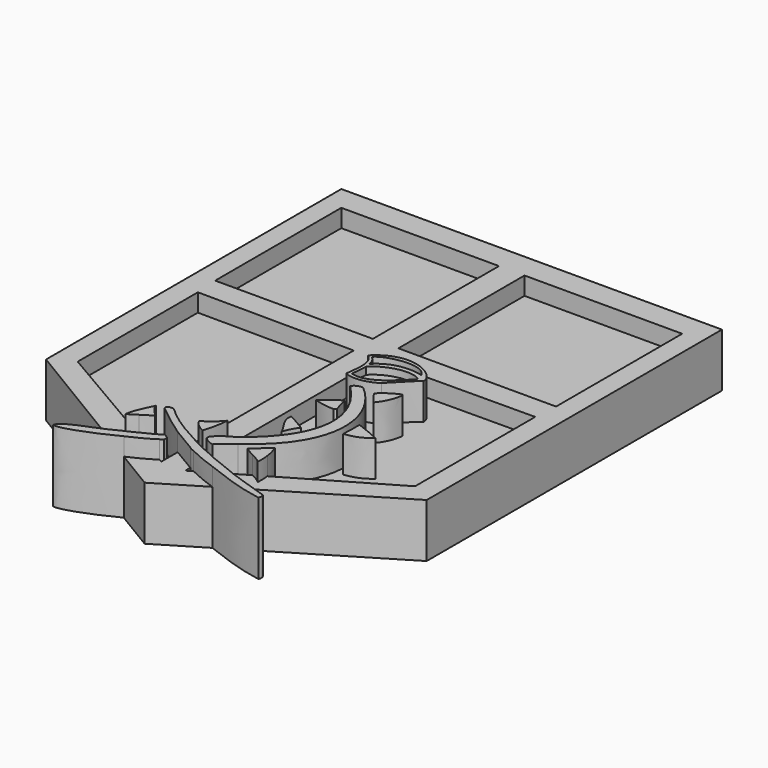
from build123d import *

# Parameters (mm, degrees)
F1_DEPTH = 3.81
F0_W     = 11.176
F0_H     = 11.176
F2_DEPTH = 2.54
F3_DEPTH = 5.08
F4_DEPTH = 4.572


with BuildPart() as f1:
    # F0 (on Top) → F1 (new body)
    with BuildSketch(Plane.XY):
        with BuildLine():
            add(Edge.make_bspline(
                [(1.7478264633, -8.0203386829), (2.3949102033, -7.7400864102), (3.0131435487, -7.4116708711), (3.5160593419, -7.0720952225)],
                knots=[0, 0, 0, 0, 2.0064429155, 2.0064429155, 2.0064429155, 2.0064429155], degree=3))
            Line((1.7478264633, -8.0203386829), (4.6047386499, -9.7420183434))
            Line((4.6047386499, -9.7420183434), (7.8442137424, -7.789792299))
            add(Edge.make_bspline(
                [(5.8583344234, -6.9758380503), (6.5180123784, -7.3072281666), (7.161768619, -7.5551345944), (7.8442137424, -7.789792299)],
                knots=[0, 0, 0, 0, 2.1462148514, 2.1462148514, 2.1462148514, 2.1462148514], degree=3))
            Line((5.8583344234, -6.9758380503), (5.4626313076, -7.2067989968))
            Line((5.4626313076, -7.2067989968), (5.4626313076, -6.7658983171))
            Line((5.4626313076, -6.7658983171), (3.7468459923, -5.7425037958))
            Line((3.7468459923, -5.7425037958), (3.7468459923, -6.668202544))
            Line((3.7468459923, -6.668202544), (3.9543234743, -6.8065118976))
            Line((3.9543234743, -6.8065118976), (3.7468459923, -6.932241008))
            Line((3.7468459923, -6.932241008), (3.7468459923, -7.2067989968))
            Line((3.7468459923, -7.2067989968), (3.5160593419, -7.0720952225))
        make_face()
        Polygon((3.7468459923, -6.668202544), (3.7468459923, -6.932241008), (3.9543234743, -6.8065118976), align=None)
    extrude(amount=F1_DEPTH)



with BuildPart() as f1b:
    # F0 (on Top) → F1, piece 2 (new body)
    with BuildSketch(Plane.XY):
        with BuildLine():
            Line((18.0921386499, 24.5479816566), (-8.8826613501, 24.5479816566))
            Line((-8.8826613501, 24.5479816566), (-8.8826613501, -1.6140183434))
            Line((-8.8826613501, -1.6140183434), (1.1086808245, -7.6351661699))
            add(Edge.make_bspline(
                [(2.9416688976, -6.7368394326), (2.373174997, -7.0127416402), (1.7493715277, -7.3646083474), (1.1086808245, -7.6351661699)],
                knots=[0, 0, 0, 0, 2.0412829797, 2.0412829797, 2.0412829797, 2.0412829797], degree=3))
            Line((2.9416688976, -6.7368394326), (0.7978946411, -5.4855777885))
            add(Edge.make_bspline(
                [(0.7978946411, -5.4855777885), (0.5607364427, -5.6443807503), (0.3392614036, -5.7966192163), (0.1594885398, -5.8946078643)],
                knots=[0.8541472288, 0.8541472288, 0.8541472288, 0.8541472288, 1.6626558138, 1.6626558138, 1.6626558138, 1.6626558138], degree=3))
            add(Edge.make_bspline(
                [(0.1594885398, -5.8946078643), (0.1844977105, -5.6643810778), (0.2451815779, -5.4372146163), (0.3267234324, -5.210568207)],
                knots=[0, 0, 0, 0, 0.730730804, 0.730730804, 0.730730804, 0.730730804], degree=3))
            Line((0.3267234324, -5.210568207), (-7.3511232622, -0.7292217924))
            Line((-7.3511232622, -0.7292217924), (-7.3511232622, 9.9187362939))
            Line((-7.3511232622, 9.9187362939), (3.7468459923, 9.8566794768))
            Line((3.7468459923, 9.8566794768), (3.7468459923, -5.1428475417))
            Line((3.7468459923, -5.1428475417), (5.4626313076, -6.1111301184))
            Line((5.4626313076, -6.1111301184), (5.4626313076, -5.3286819914))
            add(Edge.make_bspline(
                [(5.4626313076, -5.3286819914), (5.4171880556, -5.2900749749), (5.3747972554, -5.2519792783), (5.3360559978, -5.2162380889)],
                knots=[0.7997569786, 0.7997569786, 0.7997569786, 0.7997569786, 0.9823963323, 0.9823963323, 0.9823963323, 0.9823963323], degree=3))
            add(Edge.make_bspline(
                [(5.4626313076, -5.0888806677), (5.4209392766, -5.1307410959), (5.3789487872, -5.173187785), (5.3360559978, -5.2162380889)],
                knots=[1.4886530847, 1.4886530847, 1.4886530847, 1.4886530847, 1.6788346934, 1.6788346934, 1.6788346934, 1.6788346934], degree=3))
            Line((5.4626313076, -5.0888806677), (5.4626313076, 9.8566794768))
            Line((5.4626313076, 9.8566794768), (16.5606005621, 9.9187362939))
            Line((16.5606005621, 9.9187362939), (16.5606005621, -0.7292217924))
            Line((16.5606005621, -0.7292217924), (9.4219063748, -4.8958798247))
            add(Edge.make_bspline(
                [(9.4498144463, -5.7773548178), (9.4676312637, -5.4715193492), (9.4601174375, -5.1821135329), (9.4219063748, -4.8958798247)],
                knots=[0, 0, 0, 0, 0.8835893602, 0.8835893602, 0.8835893602, 0.8835893602], degree=3))
            add(Edge.make_bspline(
                [(8.7163211778, -5.3077103572), (8.9863336594, -5.4468521573), (9.2526252745, -5.5869770135), (9.4498144463, -5.7773548178)],
                knots=[0.7875820287, 0.7875820287, 0.7875820287, 0.7875820287, 1.6683513681, 1.6683513681, 1.6683513681, 1.6683513681], degree=3))
            Line((8.7163211778, -5.3077103572), (6.5198496095, -6.5897299623))
            add(Edge.make_bspline(
                [(8.467863043, -7.4139584455), (7.7391685918, -7.1327229962), (7.1244202554, -6.8972771987), (6.5198496095, -6.5897299623)],
                knots=[0, 0, 0, 0, 2.1152089565, 2.1152089565, 2.1152089565, 2.1152089565], degree=3))
            Line((8.467863043, -7.4139584455), (18.0921386499, -1.6140183434))
            Line((18.0921386499, -1.6140183434), (18.0921386499, 24.5479816566))
        make_face()
        with BuildLine():
            add(Edge.make_bspline(
                [(4.7253458761, -4.7482554801), (4.3430225924, -4.5879259706), (3.9915316738, -4.3042670004), (3.8743680343, -3.9959414862)],
                knots=[0, 0, 0, 0, 1.1358431373, 1.1358431373, 1.1358431373, 1.1358431373], degree=3))
            add(Edge.make_bspline(
                [(3.8743680343, -3.9959414862), (4.3306895532, -3.7122820504), (4.7253458761, -3.403956769), (5.0706705078, -2.9723013286)],
                knots=[0, 0, 0, 0, 1.5744773039, 1.5744773039, 1.5744773039, 1.5744773039], degree=3))
            add(Edge.make_bspline(
                [(5.0706705078, -2.9723013286), (5.0213383511, -3.5827853717), (4.9041747116, -4.1809366085), (4.7253458761, -4.7482554801)],
                knots=[0, 0, 0, 0, 1.8092159212, 1.8092159212, 1.8092159212, 1.8092159212], degree=3))
        make_face(mode=Mode.SUBTRACT)
        with Locations((-1.888773113, 17.1971733798)):
            Rectangle(F0_W, F0_H, mode=Mode.SUBTRACT)
        with Locations((11.0982504129, 17.1971733798)):
            Rectangle(F0_W, F0_H, mode=Mode.SUBTRACT)
        with BuildLine():
            add(Edge.make_bspline(
                [(5.4626313076, -5.3286819914), (5.4171880556, -5.2900749749), (5.3747972554, -5.2519792783), (5.3360559978, -5.2162380889)],
                knots=[0.7997569786, 0.7997569786, 0.7997569786, 0.7997569786, 0.9823963323, 0.9823963323, 0.9823963323, 0.9823963323], degree=3))
            Line((5.4626313076, -5.3286819914), (5.4626313076, -5.0888806677))
            add(Edge.make_bspline(
                [(5.4626313076, -5.0888806677), (5.4209392766, -5.1307410959), (5.3789487872, -5.173187785), (5.3360559978, -5.2162380889)],
                knots=[1.4886530847, 1.4886530847, 1.4886530847, 1.4886530847, 1.6788346934, 1.6788346934, 1.6788346934, 1.6788346934], degree=3))
        make_face()
    extrude(amount=F1_DEPTH)


with BuildPart() as f1_1:
    add(f1.part)

    add(f1b.part)  # F2 merges F1b
    # F0 (on Top) → F2 (join)
    with BuildSketch(Plane.XY):
        with BuildLine():
            Line((0.7978946411, -5.4855777885), (2.9416688976, -6.7368394326))
            Line((2.9416688976, -6.7368394326), (3.4156478941, -6.4474181272))
            Line((3.4156478941, -6.4474181272), (3.7468459923, -6.668202544))
            Line((3.7468459923, -6.668202544), (3.7468459923, -5.7425037958))
            add(Edge.make_bspline(
                [(3.7468459923, -5.7425037958), (2.9118994717, -5.1698186435), (2.13727355, -4.5987805352), (1.3940667268, -3.9734384045)],
                knots=[0, 0, 0, 0, 2.9436648299, 2.9436648299, 2.9436648299, 2.9436648299], degree=3))
            add(Edge.make_bspline(
                [(1.3940667268, -3.9734384045), (1.3278889237, -3.6056702957), (1.8194783479, -3.6950502545), (1.8866790924, -3.7452809047)],
                knots=[0, 0, 0, 0, 0.5428837698, 0.5428837698, 0.5428837698, 0.5428837698], degree=3))
            add(Edge.make_bspline(
                [(1.8866790924, -3.7452809047), (2.3712625261, -4.2291865684), (3.0714494642, -4.7257412225), (3.7468459923, -5.1428475417)],
                knots=[0, 0, 0, 0, 2.3266743219, 2.3266743219, 2.3266743219, 2.3266743219], degree=3))
            Line((3.7468459923, -5.1428475417), (3.7468459923, 9.8566794768))
            Line((3.7468459923, 9.8566794768), (-7.3511232622, 9.9187362939))
            Line((-7.3511232622, 9.9187362939), (-7.3511232622, -0.7292217924))
            Line((-7.3511232622, -0.7292217924), (0.3267234324, -5.210568207))
            add(Edge.make_bspline(
                [(0.3267234324, -5.210568207), (0.4654459663, -4.8249875208), (0.6645362865, -4.4409119844), (0.8510400658, -4.0458338335)],
                knots=[0.730730804, 0.730730804, 0.730730804, 0.730730804, 1.973881691, 1.973881691, 1.973881691, 1.973881691], degree=3))
            add(Edge.make_bspline(
                [(1.5713630245, -5.0165219947), (1.2786596781, -4.7041471116), (0.9113978012, -4.3504554778), (0.8510400658, -4.0458338335)],
                knots=[0, 0, 0, 0, 1.2087599726, 1.2087599726, 1.2087599726, 1.2087599726], degree=3))
            add(Edge.make_bspline(
                [(1.5713630245, -5.0165219947), (1.316488917, -5.1427171478), (1.0484399312, -5.3178107267), (0.7978946411, -5.4855777885)],
                knots=[0, 0, 0, 0, 0.8541472288, 0.8541472288, 0.8541472288, 0.8541472288], degree=3))
        make_face()
        with BuildLine():
            add(Edge.make_bspline(
                [(5.4626313076, -6.1111301184), (5.7463049889, -6.248251535), (6.1555313878, -6.4591150731), (6.5198496095, -6.5897299623)],
                knots=[0, 0, 0, 0, 1.1605034892, 1.1605034892, 1.1605034892, 1.1605034892], degree=3))
            Line((6.5198496095, -6.5897299623), (8.7163211778, -5.3077103572))
            add(Edge.make_bspline(
                [(8.0298092216, -4.9015800469), (8.2304568628, -5.0596558086), (8.4748766036, -5.1832900621), (8.7163211778, -5.3077103572)],
                knots=[0, 0, 0, 0, 0.7875820287, 0.7875820287, 0.7875820287, 0.7875820287], degree=3))
            add(Edge.make_bspline(
                [(9.1535774991, -3.8841355126), (8.725322783, -4.1867932305), (8.3324862644, -4.7373720445), (8.0298092216, -4.9015800469)],
                knots=[0, 0, 0, 0, 1.5159315689, 1.5159315689, 1.5159315689, 1.5159315689], degree=3))
            add(Edge.make_bspline(
                [(9.4219063748, -4.8958798247), (9.3772484403, -4.561353504), (9.290661138, -4.2311599671), (9.1535774991, -3.8841355126)],
                knots=[0.8835893602, 0.8835893602, 0.8835893602, 0.8835893602, 1.916255637, 1.916255637, 1.916255637, 1.916255637], degree=3))
            Line((9.4219063748, -4.8958798247), (16.5606005621, -0.7292217924))
            Line((16.5606005621, -0.7292217924), (16.5606005621, 9.9187362939))
            Line((16.5606005621, 9.9187362939), (5.4626313076, 9.8566794768))
            Line((5.4626313076, 9.8566794768), (5.4626313076, -5.0888806677))
            add(Edge.make_bspline(
                [(6.6764084622, -4.2053270154), (6.0970362861, -4.4694731571), (5.7889771144, -4.7612167258), (5.4626313076, -5.0888806677)],
                knots=[0, 0, 0, 0, 1.4886530847, 1.4886530847, 1.4886530847, 1.4886530847], degree=3))
            add(Edge.make_bspline(
                [(7.7819717117, 4.5010265894), (11.7669496685, 0.5076405359), (8.4563568234, -2.8782894369), (6.6764084622, -4.2053270154)],
                knots=[0, 0, 0, 0, 8.7762670419, 8.7762670419, 8.7762670419, 8.7762670419], degree=3))
            add(Edge.make_bspline(
                [(8.4548452869, 4.8108319752), (8.1331767142, 4.8204651102), (7.9173492268, 4.7341338359), (7.7819717117, 4.5010265894)],
                knots=[0, 0, 0, 0, 0.7407686719, 0.7407686719, 0.7407686719, 0.7407686719], degree=3))
            add(Edge.make_bspline(
                [(7.2531360202, -4.7906204127), (11.5543589927, -1.8333768239), (11.3695440814, 2.3211010266), (8.4548452869, 4.8108319752)],
                knots=[0, 0, 0, 0, 9.6763625975, 9.6763625975, 9.6763625975, 9.6763625975], degree=3))
            add(Edge.make_bspline(
                [(7.2531360202, -4.7906204127), (6.8616638891, -5.0828703679), (6.516339723, -5.3418637253), (6.18505897, -5.7105016895)],
                knots=[0, 0, 0, 0, 1.4095992865, 1.4095992865, 1.4095992865, 1.4095992865], degree=3))
            add(Edge.make_bspline(
                [(6.18505897, -5.7105016895), (5.9191426632, -5.6765978446), (5.6616221447, -5.4977377299), (5.4626313076, -5.3286819914)],
                knots=[0, 0, 0, 0, 0.7997569786, 0.7997569786, 0.7997569786, 0.7997569786], degree=3))
            Line((5.4626313076, -5.3286819914), (5.4626313076, -6.1111301184))
        make_face()
        with BuildLine():
            add(Edge.make_bspline(
                [(8.2225874066, -2.1199558396), (7.980666589, -1.5371904301), (7.3776016943, -1.06202811), (7.4968249537, -0.3716596111)],
                knots=[0, 0, 0, 0, 1.892952942, 1.892952942, 1.892952942, 1.892952942], degree=3))
            add(Edge.make_bspline(
                [(7.4968249537, -0.3716596111), (7.9144071788, -0.5795955658), (8.3382222801, -0.8238631417), (8.7610548362, -1.0945518734)],
                knots=[0, 0, 0, 0, 1.4563139836, 1.4563139836, 1.4563139836, 1.4563139836], degree=3))
            add(Edge.make_bspline(
                [(8.7610548362, -1.0945518734), (8.5307387635, -1.3888530666), (8.3580762148, -1.7526769079), (8.2225874066, -2.1199558396)],
                knots=[0, 0, 0, 0, 1.1581884418, 1.1581884418, 1.1581884418, 1.1581884418], degree=3))
        make_face(mode=Mode.SUBTRACT)
        with BuildLine():
            add(Edge.make_bspline(
                [(7.3553556576, 2.0199252758), (7.7547212131, 2.3667903151), (8.1656808034, 2.7087128256), (8.6129242554, 2.9652146623)],
                knots=[0, 0, 0, 0, 1.5732294182, 1.5732294182, 1.5732294182, 1.5732294182], degree=3))
            add(Edge.make_bspline(
                [(8.6129242554, 2.9652146623), (8.7030185387, 2.6003564708), (8.7855923921, 2.2661380935), (8.924013935, 1.8957672874)],
                knots=[0, 0, 0, 0, 1.1137748769, 1.1137748769, 1.1137748769, 1.1137748769], degree=3))
            add(Edge.make_bspline(
                [(8.924013935, 1.8957672874), (8.8682854548, 1.8838609103), (8.8227195665, 1.8443046138), (8.7929395959, 1.7774439184)],
                knots=[0, 0, 0, 0, 0.1765811486, 0.1765811486, 0.1765811486, 0.1765811486], degree=3))
            add(Edge.make_bspline(
                [(8.7929395959, 1.7774439184), (8.2995798439, 1.7669230001), (7.7650537714, 1.8754522316), (7.3553556576, 2.0199252758)],
                knots=[0, 0, 0, 0, 1.4578905268, 1.4578905268, 1.4578905268, 1.4578905268], degree=3))
        make_face(mode=Mode.SUBTRACT)
        with BuildLine():
            add(Edge.make_bspline(
                [(9.3703940511, 4.657026846), (9.526329115, 4.3411930092), (9.7634745762, 4.0558967739), (10.0183784962, 3.7871007808)],
                knots=[0, 0, 0, 0, 1.0847373876, 1.0847373876, 1.0847373876, 1.0847373876], degree=3))
            add(Edge.make_bspline(
                [(10.647803545, 5.5152899586), (10.1649090648, 5.3156521171), (9.7082797438, 5.0143827684), (9.3703940511, 4.657026846)],
                knots=[0, 0, 0, 0, 1.5389576296, 1.5389576296, 1.5389576296, 1.5389576296], degree=3))
            add(Edge.make_bspline(
                [(10.7278358191, 5.4443958215), (10.7111549005, 5.483365152), (10.6785837561, 5.5158259347), (10.647803545, 5.5152899586)],
                knots=[0, 0, 0, 0, 0.1069165262, 0.1069165262, 0.1069165262, 0.1069165262], degree=3))
            add(Edge.make_bspline(
                [(10.0183784962, 3.7871007808), (10.3937508538, 4.238513764), (10.6756044552, 4.798698239), (10.7278358191, 5.4443958215)],
                knots=[0, 0, 0, 0, 1.8027635855, 1.8027635855, 1.8027635855, 1.8027635855], degree=3))
        make_face(mode=Mode.SUBTRACT)
        with BuildLine():
            add(Edge.make_bspline(
                [(11.0556203872, -0.2232317202), (11.1070927233, 0.2977081749), (11.0771935433, 0.7693253574), (11.0852858052, 1.1983034201)],
                knots=[0, 0, 0, 0, 1.4218446441, 1.4218446441, 1.4218446441, 1.4218446441], degree=3))
            add(Edge.make_bspline(
                [(11.0852858052, 1.1983034201), (11.5990201011, 0.9836831596), (12.2310789302, 0.7833028212), (12.762288563, 0.5076405359)],
                knots=[0, 0, 0, 0, 1.813657484, 1.813657484, 1.813657484, 1.813657484], degree=3))
            add(Edge.make_bspline(
                [(12.762288563, 0.5076405359), (12.3673435301, 0.1413055725), (11.8517661467, -0.1177676531), (11.0556203872, -0.2232317202)],
                knots=[0, 0, 0, 0, 1.8565803287, 1.8565803287, 1.8565803287, 1.8565803287], degree=3))
        make_face(mode=Mode.SUBTRACT)
        with BuildLine():
            add(Edge.make_bspline(
                [(6.2449835241, 7.9964315519), (7.0174927823, 7.4354913086), (6.7296018824, 6.3399062492), (6.6649555229, 5.5675776675)],
                knots=[0, 0, 0, 0, 2.4648950629, 2.4648950629, 2.4648950629, 2.4648950629], degree=3))
            add(Edge.make_bspline(
                [(10.5703761801, 7.6710619032), (10.2531649172, 8.6557241157), (8.0357557163, 9.7695672885), (6.2449835241, 7.9964315519)],
                knots=[0, 0, 0, 0, 4.3376130576, 4.3376130576, 4.3376130576, 4.3376130576], degree=3))
            add(Edge.make_bspline(
                [(10.5871027336, 7.5067980215), (10.5815272157, 7.5615526487), (10.5759516979, 7.616307276), (10.5703761801, 7.6710619032)],
                knots=[0, 0, 0, 0, 0.1651132958, 0.1651132958, 0.1651132958, 0.1651132958], degree=3))
            add(Edge.make_bspline(
                [(8.9133325964, 5.8710686862), (9.5503591001, 6.4451182261), (10.0034726784, 7.0829736069), (10.5871027336, 7.5067980215)],
                knots=[0, 0, 0, 0, 2.3403241079, 2.3403241079, 2.3403241079, 2.3403241079], degree=3))
            add(Edge.make_bspline(
                [(6.6649555229, 5.5675776675), (6.9833141752, 5.3194463253), (8.069335483, 5.2957138978), (8.9133325964, 5.8710686862)],
                knots=[0, 0, 0, 0, 2.2687675649, 2.2687675649, 2.2687675649, 2.2687675649], degree=3))
        make_face(mode=Mode.SUBTRACT)
        with BuildLine():
            Line((5.4626313076, -7.2067989968), (5.8583344234, -6.9758380503))
            add(Edge.make_bspline(
                [(5.8583344234, -6.9758380503), (5.6914929301, -6.9214603864), (5.567043554, -6.8462723866), (5.4626313076, -6.7658983171)],
                knots=[0, 0, 0, 0, 0.4479460319, 0.4479460319, 0.4479460319, 0.4479460319], degree=3))
            Line((5.4626313076, -6.7658983171), (5.4626313076, -7.2067989968))
        make_face()
        with Locations((-1.888773113, 17.1971733798)):
            Rectangle(F0_W, F0_H)
        with Locations((11.0982504129, 17.1971733798)):
            Rectangle(F0_W, F0_H)
    extrude(amount=F2_DEPTH)

    # F0 (on Top) → F3 (join)
    with BuildSketch(Plane.XY):
        with BuildLine():
            Line((0.3267234324, -5.210568207), (0.7978946411, -5.4855777885))
            add(Edge.make_bspline(
                [(1.5713630245, -5.0165219947), (1.316488917, -5.1427171478), (1.0484399312, -5.3178107267), (0.7978946411, -5.4855777885)],
                knots=[0, 0, 0, 0, 0.8541472288, 0.8541472288, 0.8541472288, 0.8541472288], degree=3))
            add(Edge.make_bspline(
                [(1.5713630245, -5.0165219947), (1.2786596781, -4.7041471116), (0.9113978012, -4.3504554778), (0.8510400658, -4.0458338335)],
                knots=[0, 0, 0, 0, 1.2087599726, 1.2087599726, 1.2087599726, 1.2087599726], degree=3))
            add(Edge.make_bspline(
                [(0.3267234324, -5.210568207), (0.4654459663, -4.8249875208), (0.6645362865, -4.4409119844), (0.8510400658, -4.0458338335)],
                knots=[0.730730804, 0.730730804, 0.730730804, 0.730730804, 1.973881691, 1.973881691, 1.973881691, 1.973881691], degree=3))
        make_face()
        with BuildLine():
            add(Edge.make_bspline(
                [(0.7978946411, -5.4855777885), (0.5607364427, -5.6443807503), (0.3392614036, -5.7966192163), (0.1594885398, -5.8946078643)],
                knots=[0.8541472288, 0.8541472288, 0.8541472288, 0.8541472288, 1.6626558138, 1.6626558138, 1.6626558138, 1.6626558138], degree=3))
            Line((0.7978946411, -5.4855777885), (0.3267234324, -5.210568207))
            add(Edge.make_bspline(
                [(0.1594885398, -5.8946078643), (0.1844977105, -5.6643810778), (0.2451815779, -5.4372146163), (0.3267234324, -5.210568207)],
                knots=[0, 0, 0, 0, 0.730730804, 0.730730804, 0.730730804, 0.730730804], degree=3))
        make_face()
        with BuildLine():
            Line((1.7478264633, -8.0203386829), (1.1086808245, -7.6351661699))
            add(Edge.make_bspline(
                [(-2.1559654269, -9.3924161047), (-1.9764574245, -8.7245535105), (0.0426645383, -8.2730045542), (1.1086808245, -7.6351661699)],
                knots=[0, 0, 0, 0, 3.7075386013, 3.7075386013, 3.7075386013, 3.7075386013], degree=3))
            add(Edge.make_bspline(
                [(1.7478264633, -8.0203386829), (0.5305836094, -8.6686918512), (-1.6694880323, -9.5958048478), (-2.1559654269, -9.3924161047)],
                knots=[0, 0, 0, 0, 4.1378965155, 4.1378965155, 4.1378965155, 4.1378965155], degree=3))
        make_face()
        with BuildLine():
            add(Edge.make_bspline(
                [(2.9416688976, -6.7368394326), (2.373174997, -7.0127416402), (1.7493715277, -7.3646083474), (1.1086808245, -7.6351661699)],
                knots=[0, 0, 0, 0, 2.0412829797, 2.0412829797, 2.0412829797, 2.0412829797], degree=3))
            Line((1.1086808245, -7.6351661699), (1.7478264633, -8.0203386829))
            add(Edge.make_bspline(
                [(1.7478264633, -8.0203386829), (2.3949102033, -7.7400864102), (3.0131435487, -7.4116708711), (3.5160593419, -7.0720952225)],
                knots=[0, 0, 0, 0, 2.0064429155, 2.0064429155, 2.0064429155, 2.0064429155], degree=3))
            Line((3.5160593419, -7.0720952225), (2.9416688976, -6.7368394326))
        make_face()
        Polygon((3.4156478941, -6.4474181272), (2.9416688976, -6.7368394326), (3.5160593419, -7.0720952225), (3.7468459923, -6.932241008), (3.7468459923, -6.668202544), align=None)
        Polygon((5.4626313076, -6.7658983171), (5.4626313076, -6.1111301184), (3.7468459923, -5.1428475417), (3.7468459923, -5.7425037958), align=None)
        with BuildLine():
            Line((3.7468459923, -5.7425037958), (3.7468459923, -5.1428475417))
            add(Edge.make_bspline(
                [(1.8866790924, -3.7452809047), (2.3712625261, -4.2291865684), (3.0714494642, -4.7257412225), (3.7468459923, -5.1428475417)],
                knots=[0, 0, 0, 0, 2.3266743219, 2.3266743219, 2.3266743219, 2.3266743219], degree=3))
            add(Edge.make_bspline(
                [(1.3940667268, -3.9734384045), (1.3278889237, -3.6056702957), (1.8194783479, -3.6950502545), (1.8866790924, -3.7452809047)],
                knots=[0, 0, 0, 0, 0.5428837698, 0.5428837698, 0.5428837698, 0.5428837698], degree=3))
            add(Edge.make_bspline(
                [(3.7468459923, -5.7425037958), (2.9118994717, -5.1698186435), (2.13727355, -4.5987805352), (1.3940667268, -3.9734384045)],
                knots=[0, 0, 0, 0, 2.9436648299, 2.9436648299, 2.9436648299, 2.9436648299], degree=3))
        make_face()
        with BuildLine():
            Line((5.8583344234, -6.9758380503), (6.5198496095, -6.5897299623))
            add(Edge.make_bspline(
                [(5.4626313076, -6.1111301184), (5.7463049889, -6.248251535), (6.1555313878, -6.4591150731), (6.5198496095, -6.5897299623)],
                knots=[0, 0, 0, 0, 1.1605034892, 1.1605034892, 1.1605034892, 1.1605034892], degree=3))
            Line((5.4626313076, -6.1111301184), (5.4626313076, -6.7658983171))
            add(Edge.make_bspline(
                [(5.8583344234, -6.9758380503), (5.6914929301, -6.9214603864), (5.567043554, -6.8462723866), (5.4626313076, -6.7658983171)],
                knots=[0, 0, 0, 0, 0.4479460319, 0.4479460319, 0.4479460319, 0.4479460319], degree=3))
        make_face()
        with BuildLine():
            add(Edge.make_bspline(
                [(8.467863043, -7.4139584455), (9.5832124352, -7.9180570319), (10.9139792621, -8.2805417478), (12.1592897922, -8.7097994983)],
                knots=[0, 0, 0, 0, 3.9122673066, 3.9122673066, 3.9122673066, 3.9122673066], degree=3))
            Line((8.467863043, -7.4139584455), (7.8442137424, -7.789792299))
            add(Edge.make_bspline(
                [(7.8442137424, -7.789792299), (9.2654172331, -8.3500593901), (10.6636369601, -8.8590113446), (12.1592897922, -9.1123748571)],
                knots=[0, 0, 0, 0, 4.5132145903, 4.5132145903, 4.5132145903, 4.5132145903], degree=3))
            add(Edge.make_bspline(
                [(12.1592897922, -9.1123748571), (12.2802518308, -8.8921198621), (12.1696526185, -8.7476633489), (12.1592897922, -8.7097994983)],
                knots=[0, 0, 0, 0, 0.4025753587, 0.4025753587, 0.4025753587, 0.4025753587], degree=3))
        make_face()
        with BuildLine():
            Line((5.4626313076, -5.0888806677), (5.4626313076, -5.3286819914))
            add(Edge.make_bspline(
                [(6.18505897, -5.7105016895), (5.9191426632, -5.6765978446), (5.6616221447, -5.4977377299), (5.4626313076, -5.3286819914)],
                knots=[0, 0, 0, 0, 0.7997569786, 0.7997569786, 0.7997569786, 0.7997569786], degree=3))
            add(Edge.make_bspline(
                [(7.2531360202, -4.7906204127), (6.8616638891, -5.0828703679), (6.516339723, -5.3418637253), (6.18505897, -5.7105016895)],
                knots=[0, 0, 0, 0, 1.4095992865, 1.4095992865, 1.4095992865, 1.4095992865], degree=3))
            add(Edge.make_bspline(
                [(7.2531360202, -4.7906204127), (11.5543589927, -1.8333768239), (11.3695440814, 2.3211010266), (8.4548452869, 4.8108319752)],
                knots=[0, 0, 0, 0, 9.6763625975, 9.6763625975, 9.6763625975, 9.6763625975], degree=3))
            add(Edge.make_bspline(
                [(8.4548452869, 4.8108319752), (8.1331767142, 4.8204651102), (7.9173492268, 4.7341338359), (7.7819717117, 4.5010265894)],
                knots=[0, 0, 0, 0, 0.7407686719, 0.7407686719, 0.7407686719, 0.7407686719], degree=3))
            add(Edge.make_bspline(
                [(7.7819717117, 4.5010265894), (11.7669496685, 0.5076405359), (8.4563568234, -2.8782894369), (6.6764084622, -4.2053270154)],
                knots=[0, 0, 0, 0, 8.7762670419, 8.7762670419, 8.7762670419, 8.7762670419], degree=3))
            add(Edge.make_bspline(
                [(6.6764084622, -4.2053270154), (6.0970362861, -4.4694731571), (5.7889771144, -4.7612167258), (5.4626313076, -5.0888806677)],
                knots=[0, 0, 0, 0, 1.4886530847, 1.4886530847, 1.4886530847, 1.4886530847], degree=3))
        make_face()
        with BuildLine():
            add(Edge.make_bspline(
                [(8.0298092216, -4.9015800469), (8.2304568628, -5.0596558086), (8.4748766036, -5.1832900621), (8.7163211778, -5.3077103572)],
                knots=[0, 0, 0, 0, 0.7875820287, 0.7875820287, 0.7875820287, 0.7875820287], degree=3))
            Line((8.7163211778, -5.3077103572), (9.4219063748, -4.8958798247))
            add(Edge.make_bspline(
                [(9.4219063748, -4.8958798247), (9.3772484403, -4.561353504), (9.290661138, -4.2311599671), (9.1535774991, -3.8841355126)],
                knots=[0.8835893602, 0.8835893602, 0.8835893602, 0.8835893602, 1.916255637, 1.916255637, 1.916255637, 1.916255637], degree=3))
            add(Edge.make_bspline(
                [(9.1535774991, -3.8841355126), (8.725322783, -4.1867932305), (8.3324862644, -4.7373720445), (8.0298092216, -4.9015800469)],
                knots=[0, 0, 0, 0, 1.5159315689, 1.5159315689, 1.5159315689, 1.5159315689], degree=3))
        make_face()
        with BuildLine():
            Line((9.4219063748, -4.8958798247), (8.7163211778, -5.3077103572))
            add(Edge.make_bspline(
                [(8.7163211778, -5.3077103572), (8.9863336594, -5.4468521573), (9.2526252745, -5.5869770135), (9.4498144463, -5.7773548178)],
                knots=[0.7875820287, 0.7875820287, 0.7875820287, 0.7875820287, 1.6683513681, 1.6683513681, 1.6683513681, 1.6683513681], degree=3))
            add(Edge.make_bspline(
                [(9.4498144463, -5.7773548178), (9.4676312637, -5.4715193492), (9.4601174375, -5.1821135329), (9.4219063748, -4.8958798247)],
                knots=[0, 0, 0, 0, 0.8835893602, 0.8835893602, 0.8835893602, 0.8835893602], degree=3))
        make_face()
        with BuildLine():
            add(Edge.make_bspline(
                [(7.4968249537, -0.3716596111), (7.9144071788, -0.5795955658), (8.3382222801, -0.8238631417), (8.7610548362, -1.0945518734)],
                knots=[0, 0, 0, 0, 1.4563139836, 1.4563139836, 1.4563139836, 1.4563139836], degree=3))
            add(Edge.make_bspline(
                [(8.2225874066, -2.1199558396), (7.980666589, -1.5371904301), (7.3776016943, -1.06202811), (7.4968249537, -0.3716596111)],
                knots=[0, 0, 0, 0, 1.892952942, 1.892952942, 1.892952942, 1.892952942], degree=3))
            add(Edge.make_bspline(
                [(8.7610548362, -1.0945518734), (8.5307387635, -1.3888530666), (8.3580762148, -1.7526769079), (8.2225874066, -2.1199558396)],
                knots=[0, 0, 0, 0, 1.1581884418, 1.1581884418, 1.1581884418, 1.1581884418], degree=3))
        make_face()
        with BuildLine():
            add(Edge.make_bspline(
                [(11.0852858052, 1.1983034201), (11.5990201011, 0.9836831596), (12.2310789302, 0.7833028212), (12.762288563, 0.5076405359)],
                knots=[0, 0, 0, 0, 1.813657484, 1.813657484, 1.813657484, 1.813657484], degree=3))
            add(Edge.make_bspline(
                [(11.0556203872, -0.2232317202), (11.1070927233, 0.2977081749), (11.0771935433, 0.7693253574), (11.0852858052, 1.1983034201)],
                knots=[0, 0, 0, 0, 1.4218446441, 1.4218446441, 1.4218446441, 1.4218446441], degree=3))
            add(Edge.make_bspline(
                [(12.762288563, 0.5076405359), (12.3673435301, 0.1413055725), (11.8517661467, -0.1177676531), (11.0556203872, -0.2232317202)],
                knots=[0, 0, 0, 0, 1.8565803287, 1.8565803287, 1.8565803287, 1.8565803287], degree=3))
        make_face()
        with BuildLine():
            add(Edge.make_bspline(
                [(8.6129242554, 2.9652146623), (8.7030185387, 2.6003564708), (8.7855923921, 2.2661380935), (8.924013935, 1.8957672874)],
                knots=[0, 0, 0, 0, 1.1137748769, 1.1137748769, 1.1137748769, 1.1137748769], degree=3))
            add(Edge.make_bspline(
                [(7.3553556576, 2.0199252758), (7.7547212131, 2.3667903151), (8.1656808034, 2.7087128256), (8.6129242554, 2.9652146623)],
                knots=[0, 0, 0, 0, 1.5732294182, 1.5732294182, 1.5732294182, 1.5732294182], degree=3))
            add(Edge.make_bspline(
                [(8.7929395959, 1.7774439184), (8.2995798439, 1.7669230001), (7.7650537714, 1.8754522316), (7.3553556576, 2.0199252758)],
                knots=[0, 0, 0, 0, 1.4578905268, 1.4578905268, 1.4578905268, 1.4578905268], degree=3))
            add(Edge.make_bspline(
                [(8.924013935, 1.8957672874), (8.8682854548, 1.8838609103), (8.8227195665, 1.8443046138), (8.7929395959, 1.7774439184)],
                knots=[0, 0, 0, 0, 0.1765811486, 0.1765811486, 0.1765811486, 0.1765811486], degree=3))
        make_face()
        with BuildLine():
            add(Edge.make_bspline(
                [(10.647803545, 5.5152899586), (10.1649090648, 5.3156521171), (9.7082797438, 5.0143827684), (9.3703940511, 4.657026846)],
                knots=[0, 0, 0, 0, 1.5389576296, 1.5389576296, 1.5389576296, 1.5389576296], degree=3))
            add(Edge.make_bspline(
                [(9.3703940511, 4.657026846), (9.526329115, 4.3411930092), (9.7634745762, 4.0558967739), (10.0183784962, 3.7871007808)],
                knots=[0, 0, 0, 0, 1.0847373876, 1.0847373876, 1.0847373876, 1.0847373876], degree=3))
            add(Edge.make_bspline(
                [(10.0183784962, 3.7871007808), (10.3937508538, 4.238513764), (10.6756044552, 4.798698239), (10.7278358191, 5.4443958215)],
                knots=[0, 0, 0, 0, 1.8027635855, 1.8027635855, 1.8027635855, 1.8027635855], degree=3))
            add(Edge.make_bspline(
                [(10.7278358191, 5.4443958215), (10.7111549005, 5.483365152), (10.6785837561, 5.5158259347), (10.647803545, 5.5152899586)],
                knots=[0, 0, 0, 0, 0.1069165262, 0.1069165262, 0.1069165262, 0.1069165262], degree=3))
        make_face()
        with BuildLine():
            add(Edge.make_bspline(
                [(3.8743680343, -3.9959414862), (4.3306895532, -3.7122820504), (4.7253458761, -3.403956769), (5.0706705078, -2.9723013286)],
                knots=[0, 0, 0, 0, 1.5744773039, 1.5744773039, 1.5744773039, 1.5744773039], degree=3))
            add(Edge.make_bspline(
                [(4.7253458761, -4.7482554801), (4.3430225924, -4.5879259706), (3.9915316738, -4.3042670004), (3.8743680343, -3.9959414862)],
                knots=[0, 0, 0, 0, 1.1358431373, 1.1358431373, 1.1358431373, 1.1358431373], degree=3))
            add(Edge.make_bspline(
                [(5.0706705078, -2.9723013286), (5.0213383511, -3.5827853717), (4.9041747116, -4.1809366085), (4.7253458761, -4.7482554801)],
                knots=[0, 0, 0, 0, 1.8092159212, 1.8092159212, 1.8092159212, 1.8092159212], degree=3))
        make_face()
        with BuildLine():
            Line((7.8442137424, -7.789792299), (8.467863043, -7.4139584455))
            add(Edge.make_bspline(
                [(8.467863043, -7.4139584455), (7.7391685918, -7.1327229962), (7.1244202554, -6.8972771987), (6.5198496095, -6.5897299623)],
                knots=[0, 0, 0, 0, 2.1152089565, 2.1152089565, 2.1152089565, 2.1152089565], degree=3))
            Line((6.5198496095, -6.5897299623), (5.8583344234, -6.9758380503))
            add(Edge.make_bspline(
                [(5.8583344234, -6.9758380503), (6.5180123784, -7.3072281666), (7.161768619, -7.5551345944), (7.8442137424, -7.789792299)],
                knots=[0, 0, 0, 0, 2.1462148514, 2.1462148514, 2.1462148514, 2.1462148514], degree=3))
        make_face()
        with BuildLine():
            add(Edge.make_bspline(
                [(10.5703761801, 7.6710619032), (10.2531649172, 8.6557241157), (8.0357557163, 9.7695672885), (6.2449835241, 7.9964315519)],
                knots=[0, 0, 0, 0, 4.3376130576, 4.3376130576, 4.3376130576, 4.3376130576], degree=3))
            add(Edge.make_bspline(
                [(6.2449835241, 7.9964315519), (7.0174927823, 7.4354913086), (6.7296018824, 6.3399062492), (6.6649555229, 5.5675776675)],
                knots=[0, 0, 0, 0, 2.4648950629, 2.4648950629, 2.4648950629, 2.4648950629], degree=3))
            add(Edge.make_bspline(
                [(6.6649555229, 5.5675776675), (6.9833141752, 5.3194463253), (8.069335483, 5.2957138978), (8.9133325964, 5.8710686862)],
                knots=[0, 0, 0, 0, 2.2687675649, 2.2687675649, 2.2687675649, 2.2687675649], degree=3))
            add(Edge.make_bspline(
                [(8.9133325964, 5.8710686862), (9.5503591001, 6.4451182261), (10.0034726784, 7.0829736069), (10.5871027336, 7.5067980215)],
                knots=[0, 0, 0, 0, 2.3403241079, 2.3403241079, 2.3403241079, 2.3403241079], degree=3))
            add(Edge.make_bspline(
                [(10.5871027336, 7.5067980215), (10.5815272157, 7.5615526487), (10.5759516979, 7.616307276), (10.5703761801, 7.6710619032)],
                knots=[0, 0, 0, 0, 0.1651132958, 0.1651132958, 0.1651132958, 0.1651132958], degree=3))
        make_face()
        with BuildLine():
            add(Edge.make_bspline(
                [(6.920655258, 5.7281441987), (8.0938367173, 5.3621665575), (9.2400712892, 6.4729838632), (10.1884426549, 7.4827349745)],
                knots=[0, 0, 0, 0, 3.7090461391, 3.7090461391, 3.7090461391, 3.7090461391], degree=3))
            add(Edge.make_bspline(
                [(7.0229883007, 6.8689563641), (6.9888772865, 6.4886856423), (6.9547662722, 6.1084149205), (6.920655258, 5.7281441987)],
                knots=[0, 0, 0, 0, 1.1453927049, 1.1453927049, 1.1453927049, 1.1453927049], degree=3))
            add(Edge.make_bspline(
                [(10.1884426549, 7.4827349745), (9.606493637, 8.0518024042), (7.8594367951, 7.787889801), (7.0229883007, 6.8689563641)],
                knots=[0, 0, 0, 0, 3.2244108688, 3.2244108688, 3.2244108688, 3.2244108688], degree=3))
        make_face(mode=Mode.SUBTRACT)
        with BuildLine():
            add(Edge.make_bspline(
                [(6.5284371376, 7.9715549946), (6.7425146699, 7.808286231), (6.908447016, 7.5749433599), (6.9508675176, 7.2412984006)],
                knots=[0, 0, 0, 0, 0.843636248, 0.843636248, 0.843636248, 0.843636248], degree=3))
            add(Edge.make_bspline(
                [(6.5284371376, 7.9715549946), (6.8824472837, 8.5337990895), (9.4504933804, 9.1696511954), (10.0306812674, 7.9903779551)],
                knots=[0, 0, 0, 0, 3.5022947118, 3.5022947118, 3.5022947118, 3.5022947118], degree=3))
            add(Edge.make_bspline(
                [(10.0306812674, 7.9903779551), (9.2659117654, 8.2060731947), (7.9174006048, 8.248584301), (6.9508675176, 7.2412984006)],
                knots=[0, 0, 0, 0, 3.1696013807, 3.1696013807, 3.1696013807, 3.1696013807], degree=3))
        make_face(mode=Mode.SUBTRACT)
    extrude(amount=F3_DEPTH)

    # F0 (on Top) → F4 (join)
    with BuildSketch(Plane.XY):
        with BuildLine():
            add(Edge.make_bspline(
                [(7.0229883007, 6.8689563641), (6.9888772865, 6.4886856423), (6.9547662722, 6.1084149205), (6.920655258, 5.7281441987)],
                knots=[0, 0, 0, 0, 1.1453927049, 1.1453927049, 1.1453927049, 1.1453927049], degree=3))
            add(Edge.make_bspline(
                [(6.920655258, 5.7281441987), (8.0938367173, 5.3621665575), (9.2400712892, 6.4729838632), (10.1884426549, 7.4827349745)],
                knots=[0, 0, 0, 0, 3.7090461391, 3.7090461391, 3.7090461391, 3.7090461391], degree=3))
            add(Edge.make_bspline(
                [(10.1884426549, 7.4827349745), (9.606493637, 8.0518024042), (7.8594367951, 7.787889801), (7.0229883007, 6.8689563641)],
                knots=[0, 0, 0, 0, 3.2244108688, 3.2244108688, 3.2244108688, 3.2244108688], degree=3))
        make_face()
        with BuildLine():
            add(Edge.make_bspline(
                [(6.5284371376, 7.9715549946), (6.8824472837, 8.5337990895), (9.4504933804, 9.1696511954), (10.0306812674, 7.9903779551)],
                knots=[0, 0, 0, 0, 3.5022947118, 3.5022947118, 3.5022947118, 3.5022947118], degree=3))
            add(Edge.make_bspline(
                [(6.5284371376, 7.9715549946), (6.7425146699, 7.808286231), (6.908447016, 7.5749433599), (6.9508675176, 7.2412984006)],
                knots=[0, 0, 0, 0, 0.843636248, 0.843636248, 0.843636248, 0.843636248], degree=3))
            add(Edge.make_bspline(
                [(10.0306812674, 7.9903779551), (9.2659117654, 8.2060731947), (7.9174006048, 8.248584301), (6.9508675176, 7.2412984006)],
                knots=[0, 0, 0, 0, 3.1696013807, 3.1696013807, 3.1696013807, 3.1696013807], degree=3))
        make_face()
    extrude(amount=F4_DEPTH)


solid = f1_1.part
